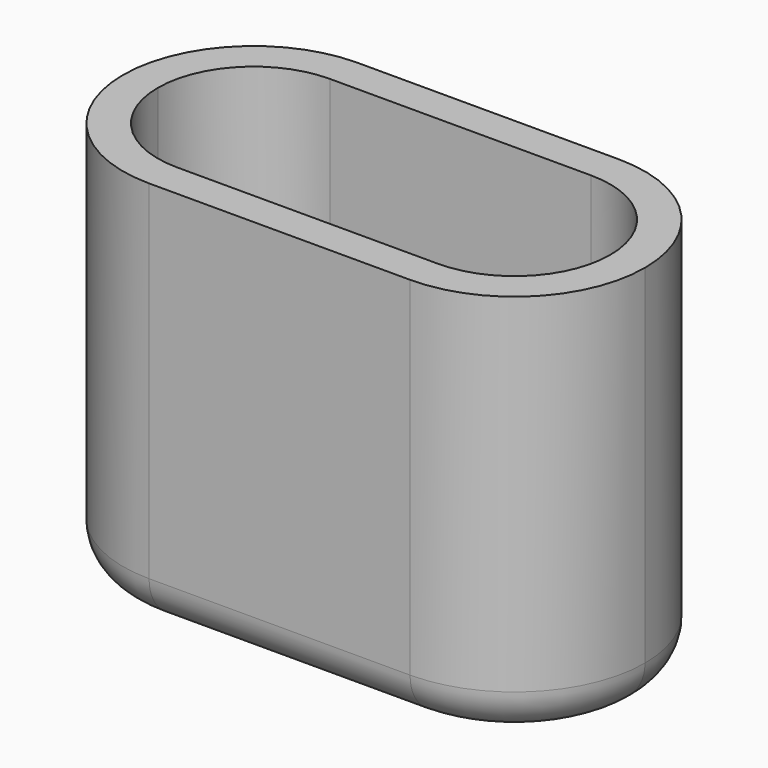
from build123d import *

# Parameters (mm, degrees)
F0_W         = 12
F0_H         = 6
F0_W_2       = 10.4
F0_H_2       = 4.4
F1_DEPTH     = 9
F2_R         = 2.19999
F3_R         = 2.99999
F4_DEPTH     = 4
F5_T4_DEPTH  = 19
F5_S5_R      = 2.99999
F5_T6_DEPTH  = 11
F5_T10_DEPTH = 19
F5_S11_R     = 2.99999
F5_T12_DEPTH = 11
F5_T16_DEPTH = 19
F5_S17_R     = 2.99999
F5_T18_DEPTH = 11
F5_T22_DEPTH = 19
F5_S23_R     = 2.99999
F5_T24_DEPTH = 11
F6_R         = 1


# Not quite as in the source:
# - a fillet or chamfer that OpenCascade refuses, or shapes differently, is made with other operations: its cross-section is extruded or revolved along the edge and cut away or added
# - a fillet or chamfer is up to 0.001 mm smaller than in the source, because OpenCascade refuses the exact size


with BuildPart() as f1:
    # F0 (on Top) → F1 (new body)
    with BuildSketch(Plane.XY):
        Rectangle(F0_W, F0_H)
        Rectangle(F0_W_2, F0_H_2, mode=Mode.SUBTRACT)
    extrude(amount=F1_DEPTH)

    # F2 (radius 2.2 in the source; OpenCascade refuses exactly that, so slightly less here)
    f2_edges = [f1.edges().sort_by_distance(p)[0] for p in [
        (-5.2, 2.2, 4.5),
        (-5.2, -2.2, 4.5),
        (5.2, 2.2, 4.5),
        (5.2, -2.2, 4.5),
    ]]
    fillet(f2_edges, radius=F2_R)

    # F3 (radius 3 in the source; OpenCascade refuses exactly that, so slightly less here)
    f3_edges = [f1.edges().sort_by_distance(p)[0] for p in [
        (-6, 3, 4.5),
        (6, 3, 4.5),
        (-6, -3, 4.5),
        (6, -3, 4.5),
    ]]
    fillet(f3_edges, radius=F3_R)

    # F0 (on Top) → F4 (join)
    with BuildSketch(Plane.XY):
        Rectangle(F0_W_2, F0_H_2)
        with BuildLine():
            Line((-0.9069178574, 1), (-4.4, 1))
            Line((-4.4, 1), (-4.4, 1.4))
            Line((-4.4, 1.4), (4.4, 1.4))
            Line((4.4, 1.4), (4.4, 1))
            Line((4.4, 1), (0.9069178574, 1))
            ThreePointArc((0.9069178574, 1), (1.2342688336, 0.5468824794), (1.35, 0))
            ThreePointArc((1.35, 0), (-0.5468824794, -1.2342688336), (-0.9069178574, 1))
        make_face(mode=Mode.SUBTRACT)
    extrude(amount=F4_DEPTH)

    # F5: fillet of radius 3 on 4 edges, made by hand


with BuildPart() as f5_tool2:
    # F5_s3 → F5_t4 (new body)
    with BuildSketch(Plane.XY.offset(-7.5)):
        with BuildLine():
            ThreePointArc((-2.2, -2.2), (-4.3213203436, -1.3213203436), (-5.2, 0.8))
            Line((-5.2, 0.8), (-5.2, -2.2))
            Line((-5.2, -2.2), (-2.2, -2.2))
        make_face()
    extrude(amount=F5_T4_DEPTH)

    # F5_s5 → F5_t6 (cut, symmetric)
    with BuildSketch(Plane.XY.offset(2)):
        with Locations((-3.00001, -1e-05)):
            Circle(F5_S5_R)
    extrude(amount=F5_T6_DEPTH, both=True, mode=Mode.SUBTRACT)


with BuildPart() as f1_1:
    add(f1.part)

    # F5_t1: cut F5_tool2
    add(f5_tool2.part, mode=Mode.SUBTRACT)


with BuildPart() as f5_tool8:
    # F5_s9 → F5_t10 (new body)
    with BuildSketch(Plane.XY.offset(-7.5)):
        with BuildLine():
            ThreePointArc((5.2, 0.8), (4.3213203436, -1.3213203436), (2.2, -2.2))
            Line((2.2, -2.2), (5.2, -2.2))
            Line((5.2, -2.2), (5.2, 0.8))
        make_face()
    extrude(amount=F5_T10_DEPTH)

    # F5_s11 → F5_t12 (cut, symmetric)
    with BuildSketch(Plane.XY.offset(2)):
        with Locations((3.00001, -1e-05)):
            Circle(F5_S11_R)
    extrude(amount=F5_T12_DEPTH, both=True, mode=Mode.SUBTRACT)


with BuildPart() as f1_2:
    add(f1_1.part)

    # F5_t7: cut F5_tool8
    add(f5_tool8.part, mode=Mode.SUBTRACT)


with BuildPart() as f5_tool14:
    # F5_s15 → F5_t16 (new body)
    with BuildSketch(Plane.XY.offset(-7.5)):
        with BuildLine():
            ThreePointArc((-5.2, -0.8), (-4.3213203436, 1.3213203436), (-2.2, 2.2))
            Line((-2.2, 2.2), (-5.2, 2.2))
            Line((-5.2, 2.2), (-5.2, -0.8))
        make_face()
    extrude(amount=F5_T16_DEPTH)

    # F5_s17 → F5_t18 (cut, symmetric)
    with BuildSketch(Plane.XY.offset(2)):
        with Locations((-3.00001, 1e-05)):
            Circle(F5_S17_R)
    extrude(amount=F5_T18_DEPTH, both=True, mode=Mode.SUBTRACT)


with BuildPart() as f1_3:
    add(f1_2.part)

    # F5_t13: cut F5_tool14
    add(f5_tool14.part, mode=Mode.SUBTRACT)


with BuildPart() as f5_tool20:
    # F5_s21 → F5_t22 (new body)
    with BuildSketch(Plane.XY.offset(-7.5)):
        with BuildLine():
            ThreePointArc((5.2, -0.8), (4.3213203436, 1.3213203436), (2.2, 2.2))
            Line((2.2, 2.2), (5.2, 2.2))
            Line((5.2, 2.2), (5.2, -0.8))
        make_face()
    extrude(amount=F5_T22_DEPTH)

    # F5_s23 → F5_t24 (cut, symmetric)
    with BuildSketch(Plane.XY.offset(2)):
        with Locations((3.00001, 1e-05)):
            Circle(F5_S23_R)
    extrude(amount=F5_T24_DEPTH, both=True, mode=Mode.SUBTRACT)


with BuildPart() as f1_4:
    add(f1_3.part)

    # F5_t19: cut F5_tool20
    add(f5_tool20.part, mode=Mode.SUBTRACT)

    # F6
    f6_edges = [f1_4.edges().sort_by_distance(p)[0] for p in [
        (0, -3, 0),
    ]]
    fillet(f6_edges, radius=F6_R)


solid = f1_4.part
